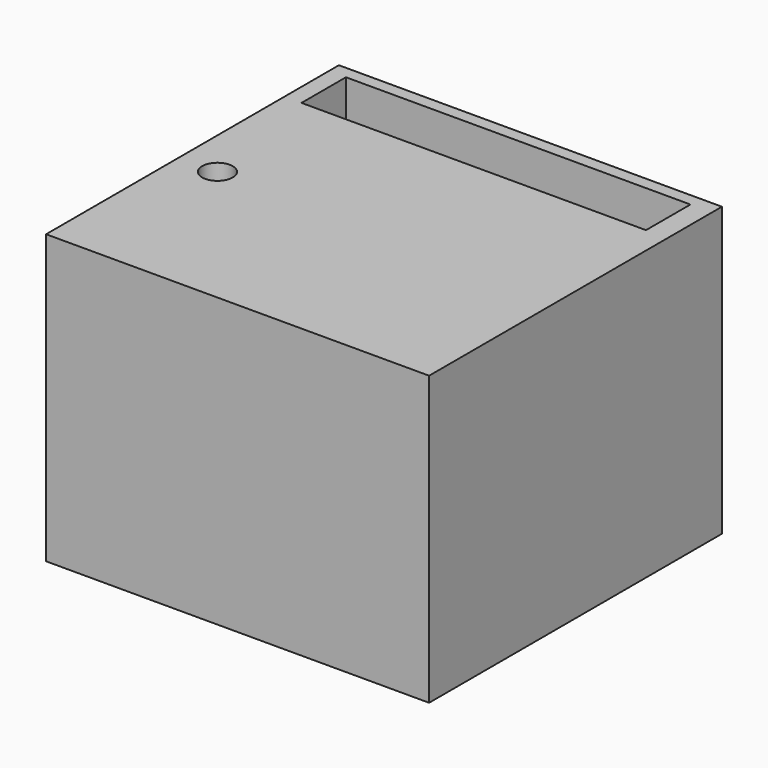
from build123d import *

# Parameters (mm, degrees)
F0_W         = 124.3373826146
F0_H         = 118.8194490969
F0_R         = 4.9797437524
F0_W_2       = 111.8300743401
F0_H_2       = 18.0252380669
F1_DEPTH     = 25.4
F2_W         = 124.3373826146
F2_H         = 118.8194490969
F2_R         = 4.9797437524
F2_W_2       = 111.8300743401
F2_H_2       = 18.0252380669
F3_DEPTH     = 68.072
F4_TEXT_SIZE = 36.156632834
F5_DEPTH     = 25.4


# Not quite as in the source:
# - Text() gives the source's letters only with a copy of the font that has no kerning and outlines rounded to 1/6400 em; it was checked with that copy


with BuildPart() as f1:
    # F0 (on Top) → F1 (new body)
    with BuildSketch(Plane.XY):
        with Locations((-6.2536559999, 5.5179279298)):
            Rectangle(F0_W, F0_H)
        with Locations((-55.9150353074, 0)):
            Circle(F0_R, mode=Mode.SUBTRACT)
        with Locations((-6.9893803447, 51.8685523421)):
            Rectangle(F0_W_2, F0_H_2, mode=Mode.SUBTRACT)
    extrude(amount=F1_DEPTH)

    # F2 (on face) → F3 (join)
    with BuildSketch(Plane.XY.offset(25.4)):
        with Locations((-6.2536559999, 5.5179279298)):
            Rectangle(F2_W, F2_H)
        with Locations((-55.9150353074, 0)):
            Circle(F2_R, mode=Mode.SUBTRACT)
        with Locations((-6.9893803447, 51.8685523421)):
            Rectangle(F2_W_2, F2_H_2, mode=Mode.SUBTRACT)
    extrude(amount=F3_DEPTH)


with BuildPart() as f5:
    # F4 (on face) → F5 (new body)
    with BuildSketch(Plane.YZ.offset(-62.9044175148)):
        with Locations((63.8020932674, -71.8097425997)):
            Text('hhhhh', F4_TEXT_SIZE, font='Open Sans', font_style=FontStyle.BOLD, text_align=(TextAlign.LEFT, TextAlign.BOTTOM))
    extrude(amount=F5_DEPTH)


solid = Compound([f1.part, f5.part])
